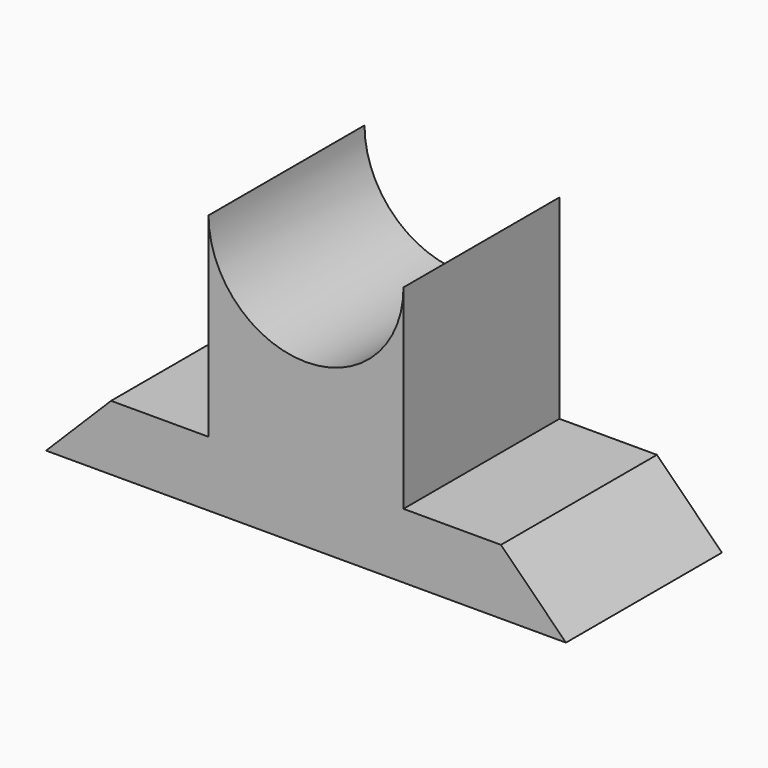
from build123d import *

# Parameters (mm, degrees)
F0_W     = 80
F0_H     = 30
F1_DEPTH = 10
F2_SIZE  = 9.99999
F4_DEPTH = 15
F5_DEPTH = 15


# Not quite as in the source:
# - a fillet or chamfer is up to 0.001 mm smaller than in the source, because OpenCascade refuses the exact size


with BuildPart() as f1:
    # F0 (on Top) → F1 (new body)
    with BuildSketch(Plane.XY):
        Rectangle(F0_W, F0_H)
    extrude(amount=F1_DEPTH)

    # F2 (size 10 in the source; OpenCascade refuses exactly that, so slightly less here)
    f2_edges = [f1.edges().sort_by_distance(p)[0] for p in [
        (-40, 0, 10),
        (40, 0, 10),
    ]]
    chamfer(f2_edges, length=F2_SIZE)

    # F3 (on Front) → F4 (join)
    with BuildSketch(Plane.XZ):
        with BuildLine():
            Line((-15, 10), (15, 10))
            Line((15, 10), (15, 40))
            ThreePointArc((15, 40), (0, 25), (-15, 40))
            Line((-15, 40), (-15, 10))
        make_face()
    extrude(amount=F4_DEPTH)

    # F5 (add): a face of the model
    f5_faces = [f1.faces().sort_by_distance(p)[0] for p in [
        (0, 0, 19.4171231702),
    ]]
    extrude(f5_faces, amount=F5_DEPTH)


solid = f1.part
